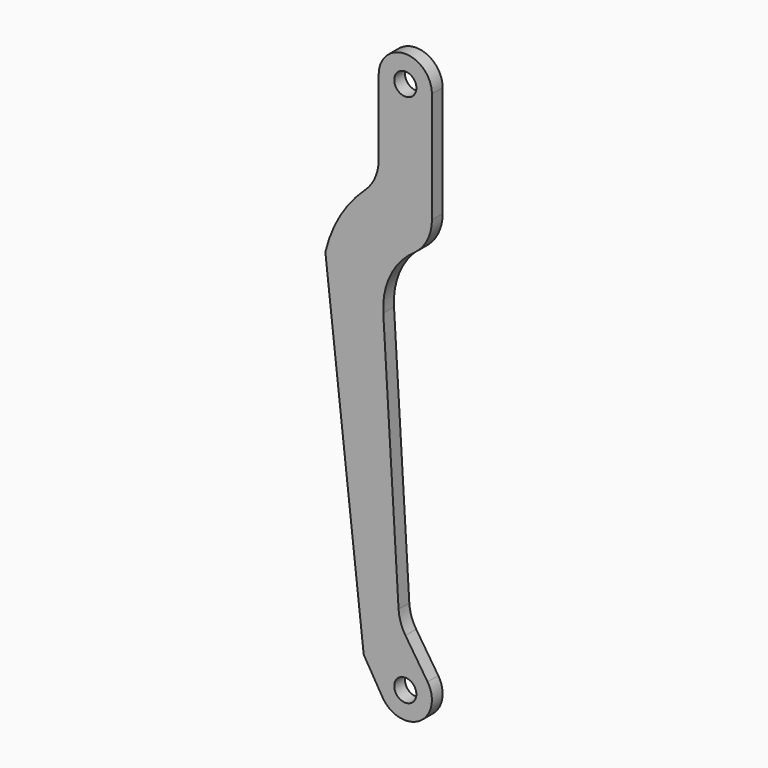
from build123d import *

# Parameters (mm, degrees)
F0_R     = 1.651
F1_DEPTH = 2


# Not quite as in the source:
# - ends of sketch curves that miss each other by under 0.0002 mm in the source are joined


with BuildPart() as f1:
    # F0 (on Front) → F1 (new body)
    with BuildSketch(Plane.XZ):
        with BuildLine():
            Line((7.937499, 23.216594), (7.937501, 39.751))
            ThreePointArc((7.937501, 39.751), (3.975101, 43.7134), (0.012701, 39.751))
            Line((0.012701, 39.751), (0.0127, 28.556342))
            ThreePointArc((0.0127, 28.556342), (-0.524833277, 25.999444372), (-2.046427009, 23.8754340098))
            ThreePointArc((-2.046427009, 23.8754340098), (-5.7457403837, 19.2987254647), (-7.9375015933, 13.8372821405))
            Line((-7.9375015933, 13.8372821405), (-2.222499, -37.1094))
            Line((-2.222499, -37.1094), (0.574712, -41.785211))
            ThreePointArc((0.574712, -41.785211), (6.0796125104, -43.1083226832), (7.2879037085, -37.5770851913))
            Line((7.2879037085, -37.5770851913), (4.000105, -32.566839))
            ThreePointArc((4.000105, -32.566839), (3.2819142622, -31.0818977846), (2.97042001, -29.4620769994))
            Line((2.97042001, -29.4620769994), (0.692124, 8.634151))
            ThreePointArc((0.692124, 8.634151), (1.7368417824, 13.9147568002), (5.2269018653, 18.0130141926))
            ThreePointArc((5.2269018653, 18.0130141926), (7.2192261395, 20.2829710591), (7.937499, 23.216594))
        make_face()
        with Locations((3.975094, -39.751)):
            Circle(F0_R, mode=Mode.SUBTRACT)
        with Locations((3.975101, 39.751)):
            Circle(F0_R, mode=Mode.SUBTRACT)
    extrude(amount=F1_DEPTH)


solid = f1.part
